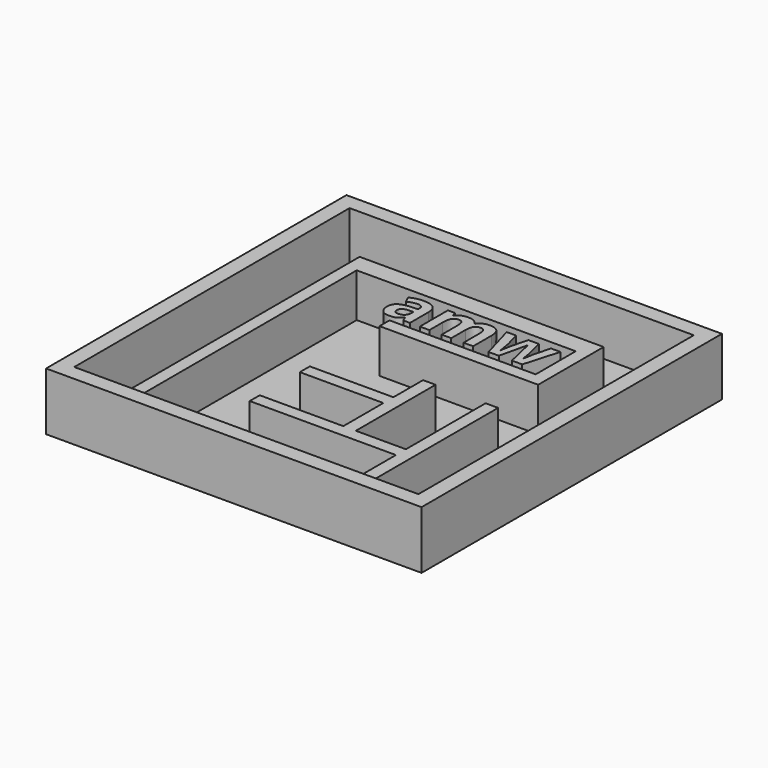
from build123d import *

# Parameters (mm, degrees)
F0_W         = 38.1
F0_H         = 38.1
F1_DEPTH     = 0.79375
F2_W         = 38.1
F2_H         = 38.1
F2_W_2       = 34.925
F2_H_2       = 34.925
F3_DEPTH     = 5.08
F4_W         = 22.225
F4_H         = 1.9555139037
F4_W_2       = 1.27
F4_W_3       = 14.8306084044
F4_H_2       = 1.27
F5_DEPTH     = 4.445
F4_R         = 1.27
F6_DEPTH     = 0.396875
F7_TEXT_SIZE = 6.5263888889
F8_DEPTH     = 4.445


# Not quite as in the source:
# - Text() gives the source's letters only with a copy of the font that has no kerning and outlines rounded to 1/6400 em; it was checked with that copy


with BuildPart() as f1:
    # F0 (on Top) → F1 (new body)
    with BuildSketch(Plane.XY):
        with Locations((1.1762361974, -14.2461048158)):
            Rectangle(F0_W, F0_H)
    extrude(amount=F1_DEPTH)

    # F2 (on face) → F3 (join)
    with BuildSketch(Plane.XY.offset(0.79375)):
        with Locations((1.1762361974, -14.2461048158)):
            Rectangle(F2_W, F2_H)
        with Locations((1.1762361974, -14.2461048158)):
            Rectangle(F2_W_2, F2_H_2, mode=Mode.SUBTRACT)
    extrude(amount=F3_DEPTH)

    # F4 (on face) → F5 (join)
    with BuildSketch(Plane.XY.offset(0.79375)):
        with Locations((1.1762361974, -2.8413617677)):
            Rectangle(F4_W, F4_H)
        Polygon((13.5587361974, -3.8191187195), (12.2887361974, -3.8191187195), (12.2887361974, -8.8991187195), (12.2887361974, -10.1691187195), (13.5587361974, -10.1691187195), align=None)
        with Locations((12.9237361974, -2.8413617677)):
            Rectangle(F4_W_2, F4_H)
        with Locations((4.8734319951, -9.5341187195)):
            Rectangle(F4_W_3, F4_H_2)
        Polygon((-11.2062638026, -1.8636048158), (-11.2062638026, -31.7086048158), (-9.9362638026, -31.7086048158), (-9.9362638026, -25.0414572656), (-9.9362638026, -20.3766748309), (-9.9362638026, -16.7861048158), (-9.9362638026, -3.8191187195), (-9.9362638026, -1.8636048158), align=None)
        Polygon((-2.5418722071, -20.2786048158), (5.9387361974, -20.2786048158), (5.9387361974, -19.0086048158), (0.8587361974, -19.0086048158), (-2.5418722071, -19.0086048158), align=None)
        Polygon((5.9387361974, -20.2786048158), (5.9387361974, -25.3586048158), (7.2087361974, -25.3586048158), (7.2087361974, -15.2491187195), (5.9387361974, -15.2491187195), (5.9387361974, -19.0086048158), align=None)
        Polygon((12.2887361974, -26.6286048158), (12.2887361974, -31.7086048158), (13.5587361974, -31.7086048158), (13.5587361974, -25.3586048158), (13.5587361974, -15.2491187195), (12.2887361974, -15.2491187195), (12.2887361974, -25.3586048158), (7.2087361974, -25.3586048158), (5.9387361974, -25.3586048158), (-2.5418722071, -25.3586048158), (-2.5418722071, -26.6286048158), align=None)
    extrude(amount=F5_DEPTH)

    # F4 (on face) → F6 (cut)
    with BuildSketch(Plane.XY.offset(0.79375)):
        with Locations((-13.7462638026, -28.0665755272)):
            Circle(F4_R)
        with Locations((8.5217421874, -29.1686048158)):
            Circle(F4_R)
    extrude(amount=-F6_DEPTH, mode=Mode.SUBTRACT)

    # F7 (on face) → F8 (join)
    with BuildSketch(Plane.XY.offset(0.79375)):
        with Locations((-4.4561937947, -8.2282980616)):
            Text('amw', F7_TEXT_SIZE, font='Open Sans', font_style=FontStyle.BOLD, text_align=(TextAlign.LEFT, TextAlign.BOTTOM))
    extrude(amount=F8_DEPTH)


solid = f1.part
